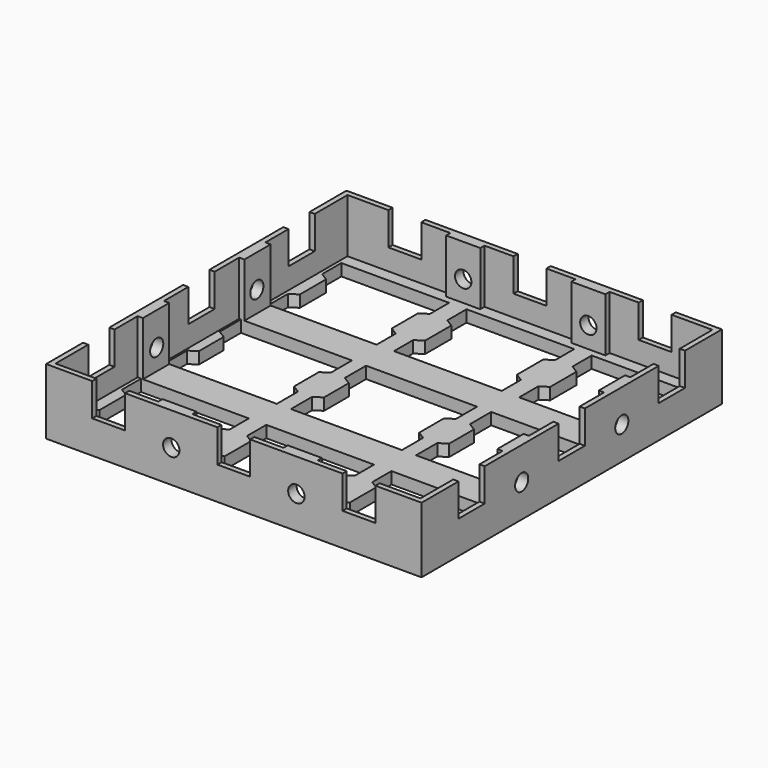
from build123d import *

# Parameters (mm, degrees)
F0_W     = 1.325
F0_H     = 2.625
F1_DEPTH = 1.8
F2_W     = 5.2
F2_H     = 0.8
F2_W_2   = 2.6
F3_DEPTH = 8.2
F2_W_3   = 0.8
F2_H_2   = 5
F2_H_3   = 2.5
F2_W_4   = 5
F2_W_5   = 2.5
F4_DEPTH = 3.2
F5_R     = 1.25
F6_DEPTH = 57.151
F7_R     = 1.25
F8_DEPTH = 57.151


# Not quite as in the source:
# - a feature names something its author has since deleted; it is built from what else it names


with BuildPart() as f1:
    # F0 (on Top) → F1 (new body)
    with BuildSketch(Plane.XY):
        Polygon((-1.325, 0), (-1.325, 2.625), (0, 2.625), (0, 57.15), (-1.325, 57.15), (-57.15, 57.15), (-57.15, 2.625), (-57.15, 0), align=None)
        Polygon((-39.425, 2.625), (-55.825, 2.625), (-55.825, 6.275), (-55.825, 12.775), (-55.825, 16.425), (-39.425, 16.425), (-39.425, 12.775), (-39.425, 6.275), align=None, mode=Mode.SUBTRACT)
        Polygon((-36.775, 16.425), (-20.375, 16.425), (-20.375, 12.775), (-20.375, 6.275), (-20.375, 2.625), (-36.775, 2.625), (-36.775, 6.275), (-36.775, 12.775), align=None, mode=Mode.SUBTRACT)
        Polygon((-1.325, 6.275), (-1.325, 2.625), (-9.525, 2.625), (-17.725, 2.625), (-17.725, 6.275), (-17.725, 12.775), (-17.725, 16.425), (-9.525, 16.425), (-1.325, 16.425), (-1.325, 12.775), align=None, mode=Mode.SUBTRACT)
        Polygon((-39.175, 31.6864380896), (-39.425, 31.5301880896), (-39.425, 25.6198119104), (-39.175, 25.4635619104), (-39.175, 21.425), (-56.075, 21.425), (-56.075, 25.4635619104), (-55.825, 25.6198119104), (-55.825, 31.5301880896), (-56.075, 31.6864380896), (-56.075, 35.725), (-39.175, 35.725), align=None, mode=Mode.SUBTRACT)
        Polygon((-39.425, 54.525), (-39.425, 50.875), (-39.425, 44.375), (-39.425, 40.725), (-55.825, 40.725), (-55.825, 44.375), (-55.825, 50.875), (-55.825, 54.525), align=None, mode=Mode.SUBTRACT)
        Polygon((-20.375, 31.5301880896), (-20.375, 25.6198119104), (-20.125, 25.4635619104), (-20.125, 21.425), (-37.025, 21.425), (-37.025, 25.4635619104), (-36.775, 25.6198119104), (-36.775, 31.5301880896), (-37.025, 31.6864380896), (-37.025, 35.725), (-20.125, 35.725), (-20.125, 31.6864380896), align=None, mode=Mode.SUBTRACT)
        Polygon((-1.075, 31.6864380896), (-1.325, 31.5301880896), (-1.325, 25.6198119104), (-1.075, 25.4635619104), (-1.075, 21.425), (-17.975, 21.425), (-17.975, 25.4635619104), (-17.725, 25.6198119104), (-17.725, 31.5301880896), (-17.975, 31.6864380896), (-17.975, 35.725), (-1.075, 35.725), align=None, mode=Mode.SUBTRACT)
        Polygon((-20.375, 50.875), (-20.375, 44.375), (-20.375, 40.725), (-36.775, 40.725), (-36.775, 44.375), (-36.775, 50.875), (-36.775, 54.525), (-20.375, 54.525), align=None, mode=Mode.SUBTRACT)
        Polygon((-17.725, 54.525), (-1.325, 54.525), (-1.325, 50.875), (-1.325, 44.375), (-1.325, 40.725), (-17.725, 40.725), (-17.725, 44.375), (-17.725, 50.875), align=None, mode=Mode.SUBTRACT)
        Polygon((-35.575, 12.025), (-36.775, 12.775), (-36.775, 6.275), (-35.575, 7.025), align=None)
        Polygon((-40.625, 7.025), (-39.425, 6.275), (-39.425, 12.775), (-40.625, 12.025), align=None)
        Polygon((-17.725, 12.775), (-17.725, 6.275), (-16.525, 7.025), (-16.525, 12.025), align=None)
        Polygon((-20.375, 6.275), (-20.375, 12.775), (-21.575, 12.025), (-21.575, 7.025), align=None)
        Polygon((-36.775, 50.875), (-36.775, 44.375), (-35.575, 45.125), (-35.575, 50.125), align=None)
        Polygon((-1.325, 44.375), (-1.325, 50.875), (-2.525, 50.125), (-2.525, 45.125), align=None)
        Polygon((-2.525, 7.025), (-1.325, 6.275), (-1.325, 12.775), (-2.525, 12.025), align=None)
        Polygon((-55.825, 12.775), (-55.825, 6.275), (-54.625, 7.025), (-54.625, 12.025), align=None)
        Polygon((-16.525, 50.125), (-17.725, 50.875), (-17.725, 44.375), (-16.525, 45.125), align=None)
        Polygon((-21.575, 45.125), (-20.375, 44.375), (-20.375, 50.875), (-21.575, 50.125), align=None)
        Polygon((-39.425, 44.375), (-39.425, 50.875), (-40.625, 50.125), (-40.625, 45.125), align=None)
        Polygon((-54.625, 50.125), (-55.825, 50.875), (-55.825, 44.375), (-54.625, 45.125), align=None)
        Polygon((-54.875, 30.9364380896), (-55.825, 31.5301880896), (-55.825, 25.6198119104), (-54.875, 26.2135619104), align=None)
        Polygon((-39.425, 25.6198119104), (-39.425, 31.5301880896), (-40.375, 30.9364380896), (-40.375, 26.2135619104), align=None)
        Polygon((-36.775, 31.5301880896), (-36.775, 25.6198119104), (-35.825, 26.2135619104), (-35.825, 30.9364380896), align=None)
        Polygon((-21.325, 26.2135619104), (-20.375, 25.6198119104), (-20.375, 31.5301880896), (-21.325, 30.9364380896), align=None)
        Polygon((-16.775, 30.9364380896), (-17.725, 31.5301880896), (-17.725, 25.6198119104), (-16.775, 26.2135619104), align=None)
        Polygon((-1.325, 25.6198119104), (-1.325, 31.5301880896), (-2.275, 30.9364380896), (-2.275, 26.2135619104), align=None)
        with Locations((-0.6625, 1.3125)):
            Rectangle(F0_W, F0_H)
    extrude(amount=F1_DEPTH)

    # F2 (on face) → F3 (join)
    with BuildSketch(Plane.XY.offset(1.8)):
        Polygon((-12.025, 56.35), (-12.025, 57.15), (-26.075, 57.15), (-26.075, 56.35), (-21.65, 56.35), (-16.45, 56.35), align=None)
        Polygon((-31.075, 56.35), (-31.075, 57.15), (-45.125, 57.15), (-45.125, 56.35), (-40.7, 56.35), (-35.5, 56.35), align=None)
        Polygon((-26.075, 0), (-12.025, 0), (-12.025, 0.8), (-16.45, 0.8), (-19.05, 0.8), (-21.65, 0.8), (-26.075, 0.8), align=None)
        Polygon((-45.125, 0), (-31.075, 0), (-31.075, 0.8), (-35.5, 0.8), (-38.1, 0.8), (-40.7, 0.8), (-45.125, 0.8), align=None)
        Polygon((-57.15, 26.075), (-57.15, 12.025), (-56.35, 12.025), (-56.35, 16.425), (-56.35, 21.425), (-56.35, 26.075), align=None)
        Polygon((-57.15, 45.125), (-57.15, 31.075), (-56.35, 31.075), (-56.35, 35.725), (-56.35, 40.725), (-56.35, 45.125), align=None)
        Polygon((-0.8, 31.075), (0, 31.075), (0, 45.125), (-0.8, 45.125), (-0.8, 40.725), (-0.8, 35.725), align=None)
        Polygon((-0.8, 12.025), (0, 12.025), (0, 26.075), (-0.8, 26.075), (-0.8, 21.425), (-0.8, 16.425), align=None)
        Polygon((-57.15, 57.15), (-57.15, 50.125), (-56.35, 50.125), (-56.35, 56.35), (-50.125, 56.35), (-50.125, 57.15), align=None)
        Polygon((-0.8, 50.125), (0, 50.125), (0, 57.15), (-7.025, 57.15), (-7.025, 56.35), (-0.8, 56.35), align=None)
        Polygon((-7.025, 0), (0, 0), (0, 7.025), (-0.8, 7.025), (-0.8, 0.8), (-7.025, 0.8), align=None)
        Polygon((-57.15, 0), (-50.125, 0), (-50.125, 0.8), (-56.35, 0.8), (-56.35, 7.025), (-57.15, 7.025), align=None)
        with Locations((-38.1, 55.95)):
            Rectangle(F2_W, F2_H)
        with Locations((-19.05, 55.95)):
            Rectangle(F2_W, F2_H)
        with Locations((-39.4, 1.2)):
            Rectangle(F2_W_2, F2_H)
        with Locations((-36.8, 1.2)):
            Rectangle(F2_W_2, F2_H)
        with Locations((-20.35, 1.2)):
            Rectangle(F2_W_2, F2_H)
        with Locations((-17.75, 1.2)):
            Rectangle(F2_W_2, F2_H)
        Polygon((-56.35, 40.725), (-56.35, 35.725), (-56.075, 35.725), (-55.55, 35.725), (-55.55, 40.725), (-55.825, 40.725), align=None)
        Polygon((-56.35, 21.425), (-56.35, 16.425), (-55.825, 16.425), (-55.55, 16.425), (-55.55, 21.425), (-56.075, 21.425), align=None)
        Polygon((-1.075, 35.725), (-0.8, 35.725), (-0.8, 40.725), (-1.325, 40.725), (-1.6, 40.725), (-1.6, 35.725), align=None)
        Polygon((-1.325, 16.425), (-0.8, 16.425), (-0.8, 21.425), (-1.075, 21.425), (-1.6, 21.425), (-1.6, 16.425), align=None)
    extrude(amount=F3_DEPTH)

    # F2 (on face) → F4 (join)
    with BuildSketch(Plane.XY.offset(1.8)):
        with Locations((-56.75, 47.625)):
            Rectangle(F2_W_3, F2_H_2)
        with Locations((-56.75, 28.575)):
            Rectangle(F2_W_3, F2_H_2)
        with Locations((-56.75, 9.525)):
            Rectangle(F2_W_3, F2_H_2)
        with Locations((-0.4, 10.775)):
            Rectangle(F2_W_3, F2_H_3)
        with Locations((-0.4, 8.275)):
            Rectangle(F2_W_3, F2_H_3)
        with Locations((-0.4, 29.825)):
            Rectangle(F2_W_3, F2_H_3)
        with Locations((-0.4, 47.625)):
            Rectangle(F2_W_3, F2_H_2)
        with Locations((-47.625, 56.75)):
            Rectangle(F2_W_4, F2_H)
        with Locations((-28.575, 56.75)):
            Rectangle(F2_W_4, F2_H)
        with Locations((-9.525, 56.75)):
            Rectangle(F2_W_4, F2_H)
        with Locations((-47.625, 0.4)):
            Rectangle(F2_W_4, F2_H)
        with Locations((-29.825, 0.4)):
            Rectangle(F2_W_5, F2_H)
        with Locations((-27.325, 0.4)):
            Rectangle(F2_W_5, F2_H)
        with Locations((-8.275, 0.4)):
            Rectangle(F2_W_5, F2_H)
        with Locations((-10.775, 0.4)):
            Rectangle(F2_W_5, F2_H)
        with Locations((-0.4, 27.325)):
            Rectangle(F2_W_3, F2_H_3)
    extrude(amount=F4_DEPTH)

    # F5 (on face) → F6 (cut, through all)
    with BuildSketch(Plane(origin=(-57.15, 0, 0), x_dir=(0, -1, 0), z_dir=(-1, 0, 0))):
        with Locations((-38.1, 5)):
            Circle(F5_R)
        with BuildLine():
            Line((-19.05, 5), (-17.8, 5))
            ThreePointArc((-17.8, 5), (-19.05, 6.25), (-20.3, 5))
            Line((-20.3, 5), (-19.05, 5))
        make_face()
        with BuildLine():
            ThreePointArc((-20.3, 5), (-19.05, 3.75), (-17.8, 5))
            Line((-17.8, 5), (-19.05, 5))
            Line((-19.05, 5), (-20.3, 5))
        make_face()
    extrude(amount=-F6_DEPTH, mode=Mode.SUBTRACT)

    # F7 (on face) → F8 (cut, through all)
    with BuildSketch(Plane.XZ):
        with BuildLine():
            Line((-19.05, 5), (-17.8, 5))
            ThreePointArc((-17.8, 5), (-19.05, 6.25), (-20.3, 5))
            Line((-20.3, 5), (-19.05, 5))
        make_face()
        with BuildLine():
            ThreePointArc((-20.3, 5), (-19.05, 3.75), (-17.8, 5))
            Line((-17.8, 5), (-19.05, 5))
            Line((-19.05, 5), (-20.3, 5))
        make_face()
        with Locations((-38.1, 5)):
            Circle(F7_R)
    extrude(amount=-F8_DEPTH, mode=Mode.SUBTRACT)


solid = f1.part
